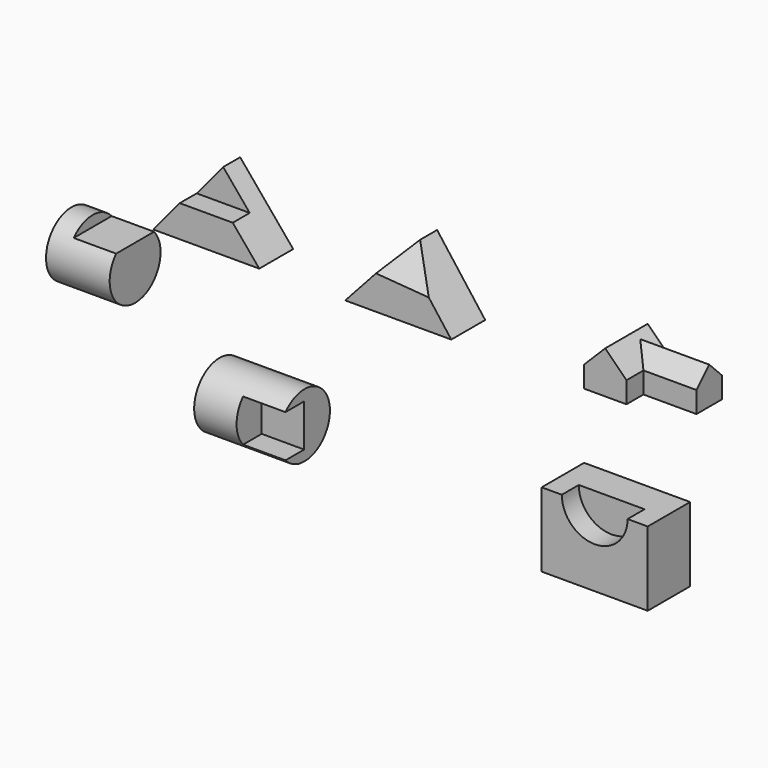
from build123d import *

# Parameters (mm, degrees)
F1_DEPTH  = 101.6
F3_DEPTH  = 50.8
F5_DEPTH  = 101.6
F9_DEPTH  = 76.2
F11_DEPTH = 127
F15_R     = 76.2
F16_DEPTH = 152.4
F18_DEPTH = 101.6
F19_R     = 76.2205995961
F20_DEPTH = 203.2
F22_DEPTH = 101.6
F23_W     = 254
F23_H     = 177.8
F24_DEPTH = 127
F26_DEPTH = 50.8


with BuildPart() as f1:
    # F0 (on Front) → F1 (new body)
    with BuildSketch(Plane.XZ):
        Polygon((127, 152.4), (0, 0), (254, 0), align=None)
    extrude(amount=-F1_DEPTH)

    # F2 (on face) → F3 (cut)
    with BuildSketch(Plane.XZ):
        Polygon((127, 152.4), (63.5, 76.2), (190.5, 76.2), align=None)
    extrude(amount=-F3_DEPTH, mode=Mode.SUBTRACT)


with BuildPart() as f5:
    # F4 (on Front) → F5 (new body)
    with BuildSketch(Plane.XZ):
        Polygon((598.7033731911, 152.4), (459.9198227574, 0), (713.9198227574, 0), align=None)
    extrude(amount=-F5_DEPTH)

    # F8 (on 3pt) → F9 (cut, symmetric)
    with BuildSketch(Plane(origin=(583.4318544266, 0, -45.1108837356), x_dir=(0, 1, 0), z_dir=(0.9970241541, 0, -0.0770897927))):
        Polygon((50.8, 198.100399998), (0, 198.100399998), (0, 121.900399998), align=None)
    extrude(amount=F9_DEPTH, both=True, mode=Mode.SUBTRACT)


with BuildPart() as f11:
    # F10 (on Front) → F11 (new body)
    with BuildSketch(Plane.XZ):
        Polygon((1032.0093378178, 50.8), (1032.0093378178, 0), (1133.6093378178, 0), (1133.6093378178, 50.8), (1082.8093697124, 101.6), align=None)
    extrude(amount=-F11_DEPTH)

    # F13 (on offset) → F14 (join, up to the next surface of F11)
    with BuildSketch(Plane.YZ.offset(1260.6093378178)):
        Polygon((50.8, 0), (127, 0), (127, 50.8), (88.9, 88.9), (50.8, 50.8), align=None)
    extrude(until=Until.NEXT, dir=(-1, 0, 0))


with BuildPart() as f16:
    # F15 (on Right) → F16 (new body)
    with BuildSketch(Plane.YZ):
        with Locations((-54.2258955538, -56.5963201225)):
            Circle(F15_R)
    extrude(amount=-F16_DEPTH)

    # F17 (on face) → F18 (cut)
    with BuildSketch(Plane.YZ):
        with BuildLine():
            ThreePointArc((2.5702310747, -5.7963201225), (-54.2258955538, 19.6036798775), (-111.0220221823, -5.7963201225))
            Line((-111.0220221823, -5.7963201225), (2.5702310747, -5.7963201225))
        make_face()
    extrude(amount=-F18_DEPTH, mode=Mode.SUBTRACT)


with BuildPart() as f20:
    # F19 (on Right) → F20 (new body)
    with BuildSketch(Plane.YZ):
        with Locations((198.8455802202, -427.576482296)):
            Circle(F19_R)
    extrude(amount=F20_DEPTH)

    # F21 (on face) → F22 (cut)
    with BuildSketch(Plane.YZ.offset(203.2)):
        with BuildLine():
            Line((197.8834101577, -376.7970818921), (142.0034101577, -376.7970818921))
            ThreePointArc((142.0034101577, -376.7970818921), (122.6249856325, -427.6041135831), (142.0402419193, -478.3970818921))
            Line((142.0402419193, -478.3970818921), (197.8834101577, -478.3970818921))
            Line((197.8834101577, -478.3970818921), (197.8834101577, -376.7970818921))
        make_face()
    extrude(amount=-F22_DEPTH, mode=Mode.SUBTRACT)


with BuildPart() as f24:
    # F23 (on Front) → F24 (new body)
    with BuildSketch(Plane.XZ):
        with Locations((1057.4588435119, -329.9870565534)):
            Rectangle(F23_W, F23_H)
    extrude(amount=-F24_DEPTH)

    # F25 (on face) → F26 (cut)
    with BuildSketch(Plane.XZ):
        with BuildLine():
            ThreePointArc((978.7019110825, -241.0870565534), (1057.4588435119, -319.8439889828), (1136.2157759414, -241.0870565534))
            Line((1136.2157759414, -241.0870565534), (978.7019110825, -241.0870565534))
        make_face()
    extrude(amount=-F26_DEPTH, mode=Mode.SUBTRACT)


solid = Compound([f1.part, f5.part, f11.part, f16.part, f20.part, f24.part])
